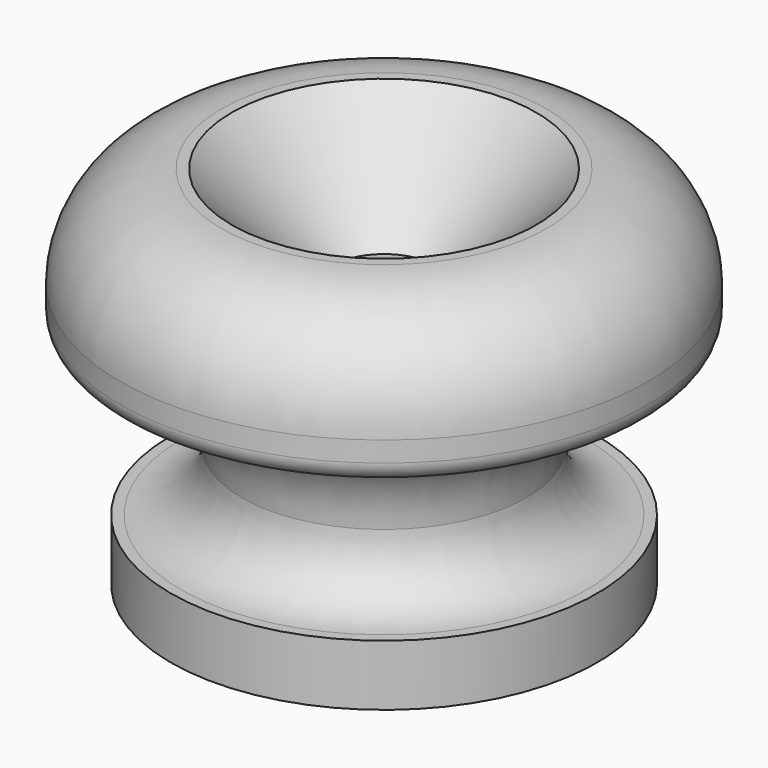
from build123d import *

# Parameters (mm, degrees)
F2_SIZE = 5
F3_R    = 0.99999


# Not quite as in the source:
# - a fillet or chamfer is up to 0.001 mm smaller than in the source, because OpenCascade refuses the exact size


with BuildPart() as f1:
    # F0 (on Front) → F1 (revolve)
    with BuildSketch(Plane.XZ):
        with BuildLine():
            Line((-2.5, -3), (-2.5, 0))
            Line((-2.5, 0), (-2.5, 15))
            Line((-2.5, 15), (-8, 15))
            ThreePointArc((-8, 15), (-11.5355339059, 13.5355339059), (-13, 10))
            Line((-13, 10), (-13, 8))
            Line((-13, 8), (-12, 8))
            ThreePointArc((-12, 8), (-8.4644660941, 6.5355339059), (-7, 3))
            ThreePointArc((-7, 3), (-7.8786796564, 0.8786796564), (-10, 0))
            Line((-10, 0), (-10.5, 0))
            Line((-10.5, 0), (-10.5, -3))
            Line((-10.5, -3), (-2.5, -3))
        make_face()
    revolve(axis=Axis((0, 0, 3.244361095), (0, 0, -1)))

    # F2
    f2_edges = [f1.edges().sort_by_distance(p)[0] for p in [
        (2.5, 0, 15),
    ]]
    chamfer(f2_edges, length=F2_SIZE)

    # F3 (radius 1 in the source; OpenCascade refuses exactly that, so slightly less here)
    f3_edges = [f1.edges().sort_by_distance(p)[0] for p in [
        (13, 0, 8),
    ]]
    fillet(f3_edges, radius=F3_R)


solid = f1.part
